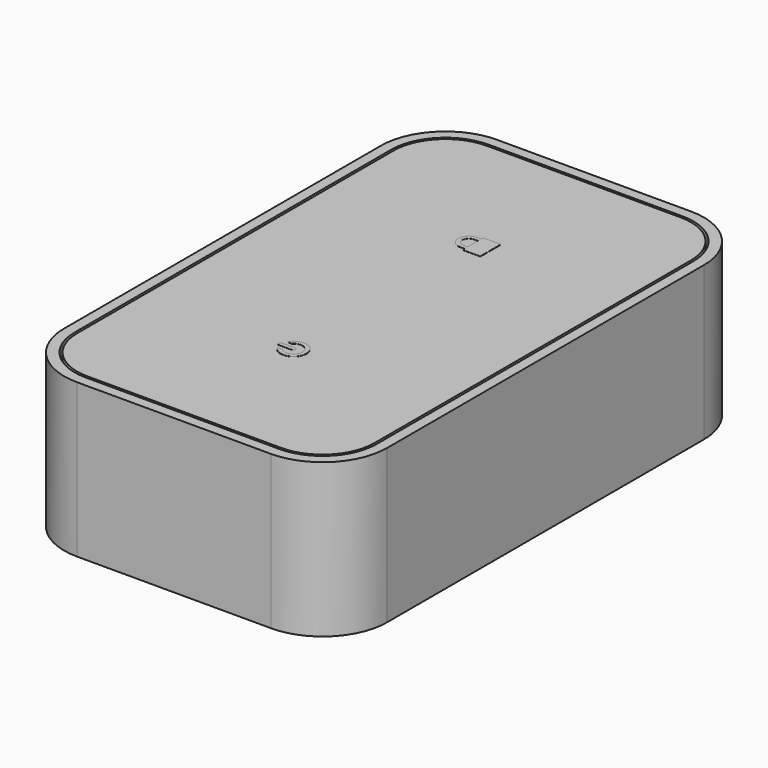
from build123d import *

# Parameters (mm, degrees)
F0_W      = 50.8
F0_H      = 82.55
F1_DEPTH  = 24.13
F2_R      = 10.16
F3_T      = -1.651
F5_DEPTH  = 6.35
F8_T      = -1.524
F14_DEPTH = 1.651
F16_DEPTH = 0.0254
F18_DEPTH = 0.0254
F19_W     = 55.88
F19_H     = 17.78
F20_DEPTH = 25.401
F21_R     = 2.54
F23_DEPTH = 1.524
F24_W     = 15.494
F24_H     = 12.7
F24_W_2   = 9.144
F24_H_2   = 3.429
F24_R     = 0.762
F25_DEPTH = 50.801
F26_R     = 1.016


with BuildPart() as f1:
    # F0 (on Top) → F1 (new body)
    with BuildSketch(Plane.XY):
        Rectangle(F0_W, F0_H)
    extrude(amount=F1_DEPTH)

    # F2
    f2_edges = [f1.edges().sort_by_distance(p)[0] for p in [
        (25.4, -41.275, 12.065),
        (-25.4, -41.275, 12.065),
        (25.4, 41.275, 12.065),
        (-25.4, 41.275, 12.065),
    ]]
    fillet(f2_edges, radius=F2_R)

    # F3
    f3_openings = [f1.faces().sort_by_distance(p)[0] for p in [
        (0, 0, 24.13),
    ]]
    offset(amount=F3_T, openings=f3_openings)

    # F19 (on Right) → F20 (cut, through all)
    with BuildSketch(Plane.YZ):
        with Locations((0, 12.065)):
            Rectangle(F19_W, F19_H)
    extrude(amount=-F20_DEPTH, mode=Mode.SUBTRACT)

    # F21
    f21_edges = [f1.edges().sort_by_distance(p)[0] for p in [
        (-24.5745, 27.94, 20.955),
        (-24.5745, -27.94, 20.955),
        (-24.5745, -27.94, 3.175),
        (-24.5745, 27.94, 3.175),
    ]]
    fillet(f21_edges, radius=F21_R)


with BuildPart() as f5:
    # F4 (on face) → F5 (new body)
    with BuildSketch(Plane.XY.offset(24.13)):
        with BuildLine():
            Line((15.24, 39.243), (-15.24, 39.243))
            ThreePointArc((-15.24, 39.243), (-20.9873639175, 36.8623639175), (-23.368, 31.115))
            Line((-23.368, 31.115), (-23.368, -31.115))
            ThreePointArc((-23.368, -31.115), (-20.9873639175, -36.8623639175), (-15.24, -39.243))
            Line((-15.24, -39.243), (15.24, -39.243))
            ThreePointArc((15.24, -39.243), (20.9873639175, -36.8623639175), (23.368, -31.115))
            Line((23.368, -31.115), (23.368, 31.115))
            ThreePointArc((23.368, 31.115), (20.9873639175, 36.8623639175), (15.24, 39.243))
        make_face()
    extrude(amount=-F5_DEPTH)

    # F8
    f8_openings = [f5.faces().sort_by_distance(p)[0] for p in [
        (0, 0, 17.78),
        (0, -39.243, 20.955),
        (20.987364, -36.862364, 20.955),
        (-20.987364, -36.862364, 20.955),
        (23.368, 0, 20.955),
        (20.987364, 36.862364, 20.955),
        (0, 39.243, 20.955),
        (-20.987364, 36.862364, 20.955),
        (-23.368, 0, 20.955),
    ]]
    offset(amount=F8_T, openings=f8_openings)


with BuildPart() as f14:
    # F13 (on offset) → F14 (new body)
    with BuildSketch(Plane(origin=(0, 0, 19.558), x_dir=(1, 0, 0), z_dir=(0, 0, -1))):
        with BuildLine():
            Line((-20.828, 31.115), (-20.828, -31.115))
            ThreePointArc((-20.828, -31.115), (-19.1913126933, -35.0663126933), (-15.24, -36.703))
            Line((-15.24, -36.703), (15.24, -36.703))
            ThreePointArc((15.24, -36.703), (19.1913126933, -35.0663126933), (20.828, -31.115))
            Line((20.828, -31.115), (20.828, 31.115))
            ThreePointArc((20.828, 31.115), (19.1913126933, 35.0663126933), (15.24, 36.703))
            Line((15.24, 36.703), (-15.24, 36.703))
            ThreePointArc((-15.24, 36.703), (-19.1913126933, 35.0663126933), (-20.828, 31.115))
        make_face()
    extrude(amount=F14_DEPTH)


with BuildPart() as f16:
    # F15 (on face) → F16 (new body)
    with BuildSketch(Plane.XY.offset(24.13)):
        with BuildLine():
            ThreePointArc((-2.032, -18.0975), (-2.0195881687, -18.0972573032), (-2.0071953125, -18.0965295839))
            ThreePointArc((-2.0071953125, -18.0965295839), (-2.0071187349, -18.0970148012), (-2.0070420399, -18.0975))
            Line((-2.0070420399, -18.0975), (0, -18.0975))
            ThreePointArc((0, -18.0975), (0.3175, -17.78), (0, -17.4625))
            Line((0, -17.4625), (-2.0070420399, -17.4625))
            ThreePointArc((-2.0070420399, -17.4625), (-2.0071187349, -17.4629851988), (-2.0071953125, -17.4634704161))
            ThreePointArc((-2.0071953125, -17.4634704161), (-2.0195881687, -17.4627426968), (-2.032, -17.4625))
            ThreePointArc((-2.032, -17.4625), (-2.3495, -17.78), (-2.032, -18.0975))
        make_face()
        with BuildLine():
            ThreePointArc((-2.0070420399, -18.0975), (-2.0071187349, -18.0970148012), (-2.0071953125, -18.0965295839))
            ThreePointArc((-2.0071953125, -18.0965295839), (-2.0195881687, -18.0972573032), (-2.032, -18.0975))
            Line((-2.032, -18.0975), (-2.0070420399, -18.0975))
        make_face()
        with BuildLine():
            Line((-2.0070420399, -17.4625), (-2.032, -17.4625))
            ThreePointArc((-2.032, -17.4625), (-2.0195881687, -17.4627426968), (-2.0071953125, -17.4634704161))
            ThreePointArc((-2.0071953125, -17.4634704161), (-2.0071187349, -17.4629851988), (-2.0070420399, -17.4625))
        make_face()
    extrude(amount=F16_DEPTH)


with BuildPart() as f16b:
    # F15 (on face) → F16, piece 2 (new body)
    with BuildSketch(Plane.XY.offset(24.13)):
        with BuildLine():
            ThreePointArc((-0.9861117026, -16.7904583333), (1.397, -17.78), (-0.9861117026, -18.7695416667))
            ThreePointArc((-0.9861117026, -18.7695416667), (-1.0272592949, -18.7421251553), (-1.075758221, -18.7325))
            Line((-1.075758221, -18.7325), (-1.569619301, -18.7325))
            ThreePointArc((-1.569619301, -18.7325), (-1.6820220738, -18.8003847171), (-1.6742605877, -18.9314666667))
            ThreePointArc((-1.6742605877, -18.9314666667), (2.032, -17.78), (-1.6742605877, -16.6285333333))
            ThreePointArc((-1.6742605877, -16.6285333333), (-1.6820220738, -16.7596152829), (-1.569619301, -16.8275))
            Line((-1.569619301, -16.8275), (-1.075758221, -16.8275))
            ThreePointArc((-1.075758221, -16.8275), (-1.0272592949, -16.8178748447), (-0.9861117026, -16.7904583333))
        make_face()
    extrude(amount=F16_DEPTH)


with BuildPart() as f18:
    # F17 (on face) → F18 (new body)
    with BuildSketch(Plane.XY.offset(24.13)):
        with BuildLine():
            Line((2.54, 15.748), (2.54, 19.812))
            Line((2.54, 19.812), (-0.254, 19.812))
            Line((-0.254, 19.812), (-0.254, 19.431))
            Line((-0.254, 19.431), (-0.889, 19.431))
            ThreePointArc((-0.889, 19.431), (-2.54, 17.78), (-0.889, 16.129))
            Line((-0.889, 16.129), (-0.254, 16.129))
            Line((-0.254, 16.129), (-0.254, 15.748))
            Line((-0.254, 15.748), (2.54, 15.748))
        make_face()
        with BuildLine():
            ThreePointArc((-0.889, 16.764), (-1.905, 17.78), (-0.889, 18.796))
            Line((-0.889, 18.796), (-0.254, 18.796))
            Line((-0.254, 18.796), (-0.254, 16.764))
            Line((-0.254, 16.764), (-0.889, 16.764))
        make_face(mode=Mode.SUBTRACT)
    extrude(amount=F18_DEPTH)


with BuildPart() as f23:
    # F22 (on face) → F23 (new body)
    with BuildSketch(Plane(origin=(-25.4, 0, 0), x_dir=(0, -1, 0), z_dir=(-1, 0, 0))):
        with BuildLine():
            ThreePointArc((25.4, 3.429), (27.0164461018, 4.0985538982), (27.686, 5.715))
            Line((27.686, 5.715), (27.686, 18.415))
            ThreePointArc((27.686, 18.415), (27.0164461018, 20.0314461018), (25.4, 20.701))
            Line((25.4, 20.701), (-25.4, 20.701))
            ThreePointArc((-25.4, 20.701), (-27.0164461018, 20.0314461018), (-27.686, 18.415))
            Line((-27.686, 18.415), (-27.686, 5.715))
            ThreePointArc((-27.686, 5.715), (-27.0164461018, 4.0985538982), (-25.4, 3.429))
            Line((-25.4, 3.429), (25.4, 3.429))
        make_face()
    extrude(amount=-F23_DEPTH)

    # F24 (on face) → F25 (cut, through all)
    with BuildSketch(Plane(origin=(-25.4, 0, 0), x_dir=(0, -1, 0), z_dir=(-1, 0, 0))):
        with Locations((-17.145, 12.065)):
            Rectangle(F24_W, F24_H)
        with Locations((0.889, 12.065)):
            Rectangle(F24_W, F24_H)
        with Locations((20.574, 16.3195)):
            Rectangle(F24_W_2, F24_H_2)
        with Locations((12.235950573, 17.1858270001)):
            Circle(F24_R)
    extrude(amount=-F25_DEPTH, mode=Mode.SUBTRACT)

    # F26
    f26_edges = [f23.edges().sort_by_distance(p)[0] for p in [
        (-24.638, -16.002, 18.034),
        (-24.638, -25.146, 18.034),
        (-24.638, -16.002, 14.605),
        (-24.638, -25.146, 14.605),
    ]]
    fillet(f26_edges, radius=F26_R)


solid = Compound([f1.part, f5.part, f14.part, f16.part, f16b.part, f18.part, f23.part])
